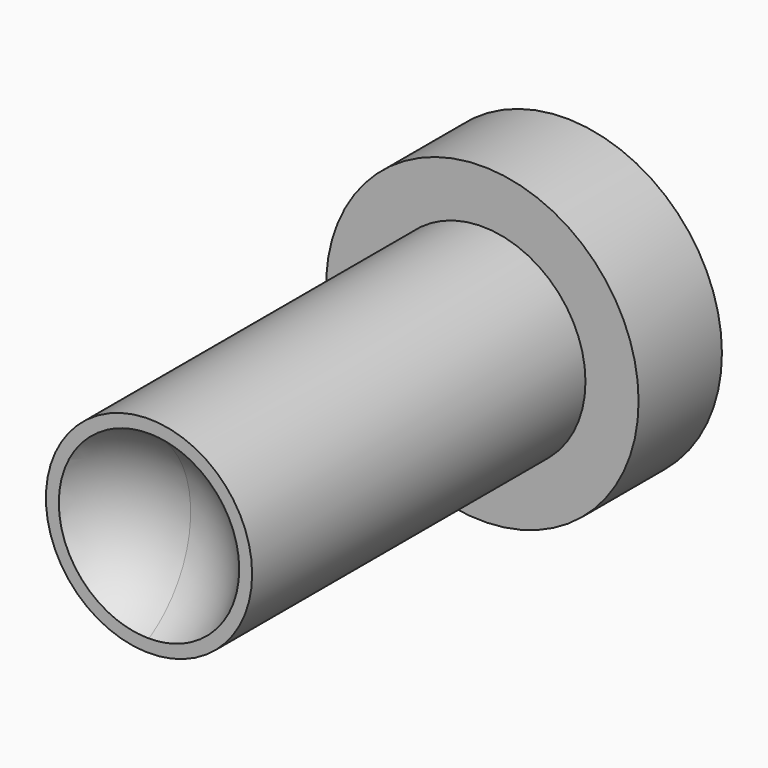
from build123d import *
from build123d import SkipClean  # not in build123d's __all__

# Parameters (mm, degrees)
F0_R     = 19.05
F1_DEPTH = 12.7
F2_R     = 12.573
F3_DEPTH = 50.8


with BuildPart() as f1:
    # F0 (on Front) → F1 (new body)
    with BuildSketch(Plane.XZ):
        Circle(F0_R)
    extrude(amount=F1_DEPTH)

    # F2 (on face) → F3 (join)
    with BuildSketch(Plane.XZ.offset(12.7)):
        Circle(F2_R)
    extrude(amount=F3_DEPTH)

    # F4 (on Right) → F5 (revolve, cut)
    with BuildSketch(Plane.YZ):
        with BuildLine():
            ThreePointArc((-69.85, -12.7), (-57.15, 0), (-69.85, 12.7))
            Line((-69.85, 12.7), (-69.85, -12.7))
        make_face()
    with SkipClean():  # cleaning this boolean's faces spoils the solid; the shape is the same uncleaned
        revolve(axis=Axis((0, -69.85, 0), (0, 0, -1)), mode=Mode.SUBTRACT)


solid = f1.part
